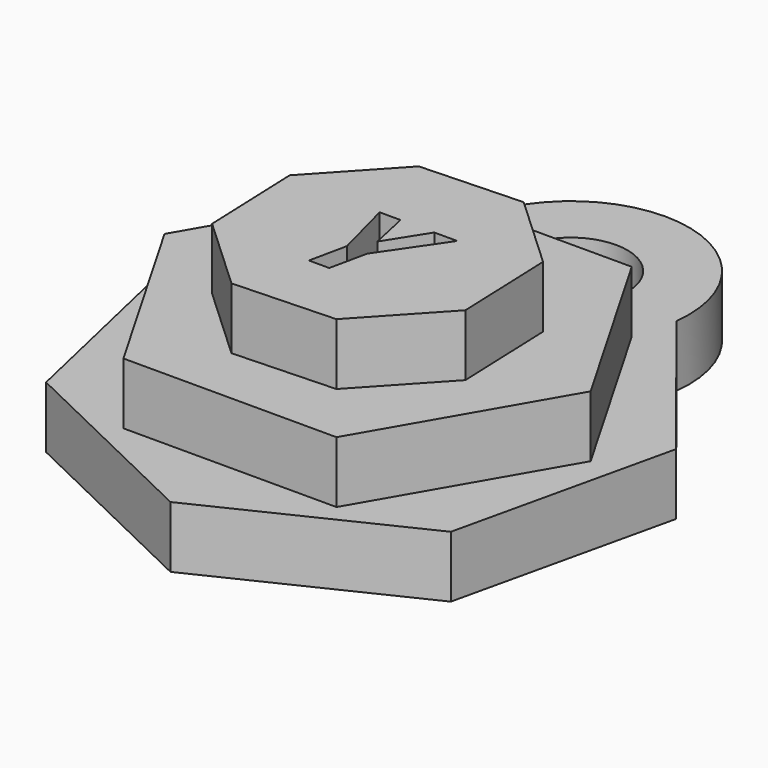
from build123d import *

# Parameters (mm, degrees)
F1_DEPTH     = 6.35
F3_DEPTH     = 6.35
F5_DEPTH     = 6.35
F6_TEXT_SIZE = 14.1953208773
F7_DEPTH     = 6.35
F8_R         = 12.1995857704
F8_R_2       = 5.8383936039
F9_DEPTH     = 6.35


# Not quite as in the source:
# - Text() gives the source's letters only with a copy of the font that has no kerning and outlines rounded to 1/6400 em; it was checked with that copy


with BuildPart() as f1:
    # F0 (on Top) → F1 (new body)
    with BuildSketch(Plane.XY):
        Polygon((0, -26.7232151235), (20.8930508963, -16.6616521024), (26.0532083271, 5.9464747876), (11.594768499, 24.0767848765), (-11.594768499, 24.0767848765), (-26.0532083271, 5.9464747876), (-20.8930508963, -16.6616521024), align=None)
    extrude(amount=F1_DEPTH)

    # F2 (on face) → F3 (join)
    with BuildSketch(Plane.XY.offset(6.35)):
        Polygon((-10.9985226281, -19.05), (10.9985226281, -19.05), (21.9970452561, 0), (10.9985226281, 19.05), (-10.9985226281, 19.05), (-21.9970452561, 0), align=None)
    extrude(amount=F3_DEPTH)

    # F4 (on face) → F5 (join)
    with BuildSketch(Plane.XY.offset(12.7)):
        Polygon((5.7401583154, -12.4905392824), (12.8910498971, -4.7732401574), (12.4905392824, 5.7401583154), (4.7732401574, 12.8910498971), (-5.7401583154, 12.4905392824), (-12.8910498971, 4.7732401574), (-12.4905392824, -5.7401583154), (-4.7732401574, -12.8910498971), align=None)
    extrude(amount=F5_DEPTH)

    # F6 (on face) → F7 (cut)
    with BuildSketch(Plane.XY.offset(19.05)):
        with Locations((-4.4893447919, -5.8755339571)):
            Text('Y', F6_TEXT_SIZE, font='Open Sans', font_style=FontStyle.BOLDITALIC, text_align=(TextAlign.LEFT, TextAlign.BOTTOM))
    extrude(amount=-F7_DEPTH, mode=Mode.SUBTRACT)

    # F8 (on Top) → F9 (join)
    with BuildSketch(Plane.XY):
        with Locations((0, 24.9320268631)):
            Circle(F8_R)
        with Locations((0, 24.9320268631)):
            Circle(F8_R_2, mode=Mode.SUBTRACT)
    extrude(amount=F9_DEPTH)


solid = f1.part
